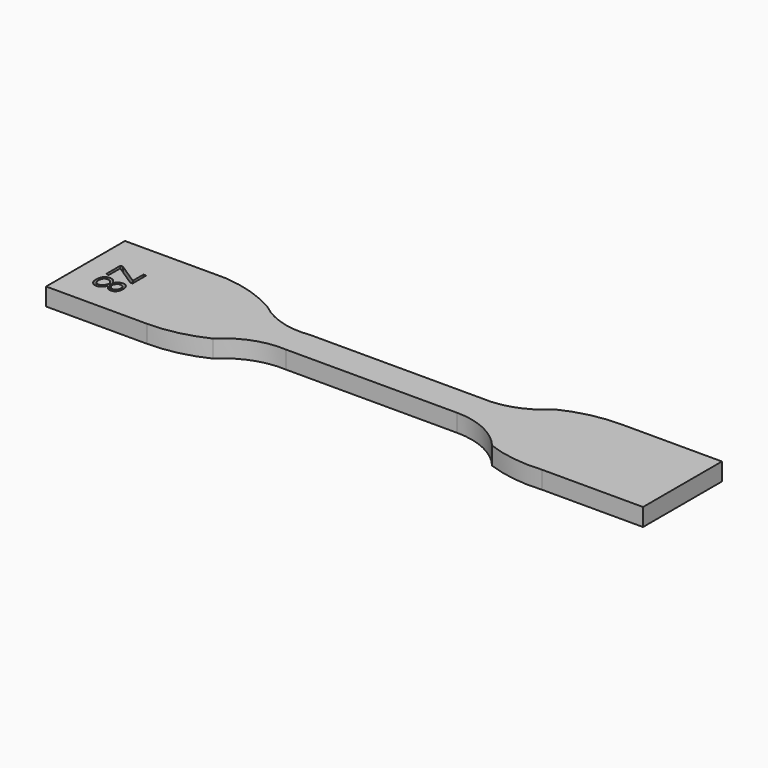
from build123d import *

# Parameters (mm, degrees)
F1_DEPTH     = 3.4
F2_TEXT_SIZE = 7.0564552314
F3_DEPTH     = 1


# Not quite as in the source:
# - Text() gives the source's letters only with a copy of the font that has no kerning and outlines rounded to 1/6400 em; it was checked with that copy


with BuildPart() as f1:
    # F0 (on Top) → F1 (new body)
    with BuildSketch(Plane.XY):
        with BuildLine():
            Line((-14.4320548165, 19.7811394548), (-33.8720548165, 19.7811394548))
            Line((-33.8720548165, 19.7811394548), (-33.8720548165, 0.7811394548))
            Line((-33.8720548165, 0.7811394548), (-14.4320548165, 0.7811394548))
            ThreePointArc((-14.4320548165, 0.7811394548), (-8.9053122052, 1.3996892086), (-3.6520548165, 3.2247301661))
            ThreePointArc((-3.6520548165, 3.2247301661), (1.3014698263, 6.4128780055), (7.1279451835, 7.2811394548))
            Line((7.1279451835, 7.2811394548), (40.1279451835, 7.2811394548))
            ThreePointArc((40.1279451835, 7.2811394548), (46.0837574042, 5.9511158081), (50.9079451835, 2.2137538538))
            ThreePointArc((50.9079451835, 2.2137538538), (56.2191047011, 0.9041953221), (61.6879451835, 0.7811394548))
            Line((61.6879451835, 0.7811394548), (81.1279451835, 0.7811394548))
            Line((81.1279451835, 0.7811394548), (81.1279451835, 19.7811394548))
            Line((81.1279451835, 19.7811394548), (61.6879451835, 19.7811394548))
            ThreePointArc((61.6879451835, 19.7811394548), (56.1612025723, 19.162589701), (50.9079451835, 17.3375487435))
            ThreePointArc((50.9079451835, 17.3375487435), (45.9544205407, 14.1494009041), (40.1279451835, 13.2811394548))
            Line((40.1279451835, 13.2811394548), (7.1279451835, 13.2811394548))
            ThreePointArc((7.1279451835, 13.2811394548), (1.4167452884, 13.6925537245), (-3.6520548165, 16.3560723447))
            ThreePointArc((-3.6520548165, 16.3560723447), (-8.8458057958, 18.686276846), (-14.4320548165, 19.7811394548))
        make_face()
    extrude(amount=F1_DEPTH)

    # F2 (on face) → F3 (cut)
    with BuildSketch(Plane.XY.offset(3.4)):
        with Locations(Location((-29.3720550835, 13.353464842), (0, 0, -90))):
            Text('Z8', F2_TEXT_SIZE, font='Open Sans', text_align=(TextAlign.LEFT, TextAlign.BOTTOM))
    extrude(amount=-F3_DEPTH, mode=Mode.SUBTRACT)


solid = f1.part
